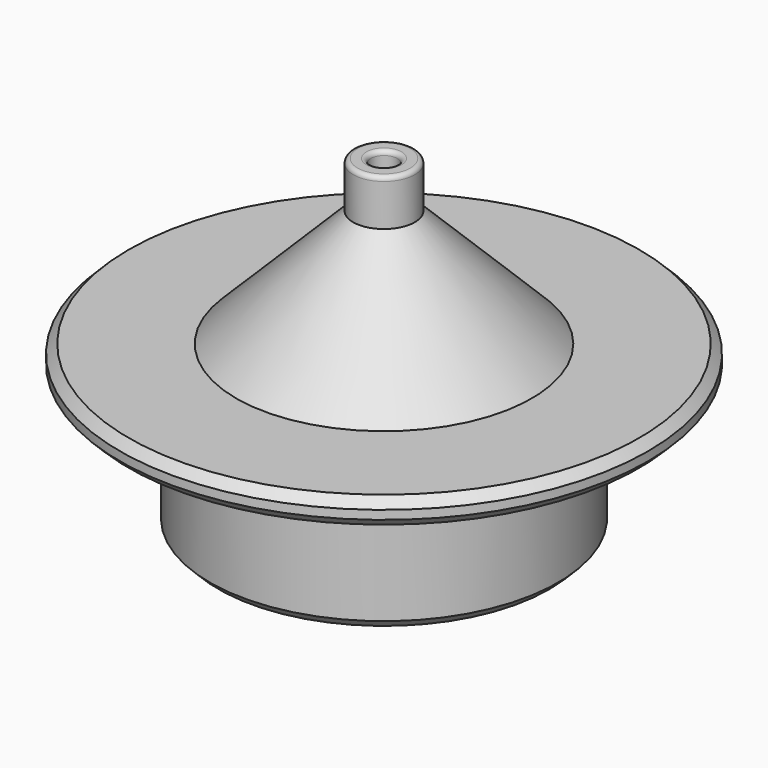
from build123d import *

# Parameters (mm, degrees)
F2_SIZE = 1
F3_R    = 0.5


# Not quite as in the source:
# - a feature names something its author has since deleted; it is built from what else it names


with BuildPart() as f1:
    # F0 (on Front) → F1 (revolve)
    with BuildSketch(Plane.XZ):
        Polygon((-19.8, 15.4426406871), (-19.8, 0), (-16.8, 0), (-16.8, 14.2), (-1, 30), (-1.5, 33), (-1.5, 37), (-3.5, 37), (-3.5, 31.7426406871), (-16.8, 18.4426406871), (-30, 18.4426406871), (-30, 15.4426406871), align=None)
    revolve(axis=Axis((0, 0, 35), (0, 0, 1)))

    # F2
    f2_edges = [f1.edges().sort_by_distance(p)[0] for p in [
        (30, 0, 18.442641),
        (30, 0, 15.442641),
        (19.8, 0, 0),
        (16.8, 0, 0),
    ]]
    chamfer(f2_edges, length=F2_SIZE)

    # F3
    f3_edges = [f1.edges().sort_by_distance(p)[0] for p in [
        (1.5, 0, 37),
        (3.5, 0, 37),
    ]]
    fillet(f3_edges, radius=F3_R)


solid = f1.part
